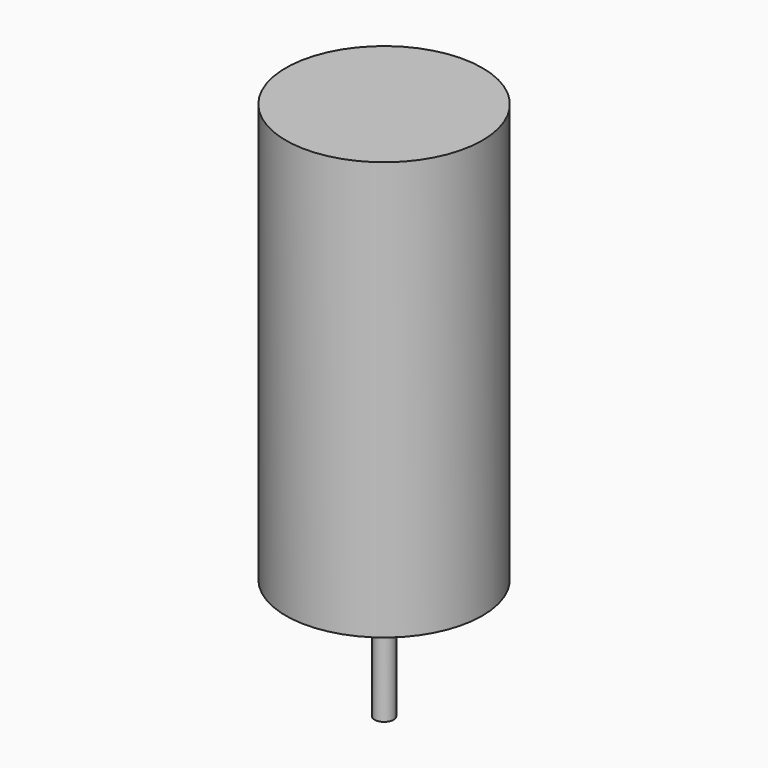
from build123d import *

# Parameters (mm, degrees)
F0_R            = 1.5
F1_DEPTH        = 19
F0_R_2          = 6
F2_DEPTH        = 3
F0_R_3          = 15.5
F3_DEPTH        = 66
F4_DEPTH        = 10
F4_COPIES_COUNT = 4


# Not quite as in the source:
# - a pattern or mirror of a feature is missing from the dataset's text; its kind, count and spacing are read off the source's solid


with BuildPart() as f1:
    # F0 (on Top) → F1 (new body)
    with BuildSketch(Plane.XY):
        Circle(F0_R)
    extrude(amount=-F1_DEPTH)

    # F0 (on Top) → F2 (join)
    with BuildSketch(Plane.XY):
        Circle(F0_R_2)
        Circle(F0_R, mode=Mode.SUBTRACT)
    extrude(amount=-F2_DEPTH)

    # F0 (on Top) → F3 (join)
    with BuildSketch(Plane.XY):
        Circle(F0_R_3)
        Circle(F0_R_2, mode=Mode.SUBTRACT)
        with Locations((7.7781745931, 7.7781745931)):
            Circle(F0_R, mode=Mode.SUBTRACT)
        Circle(F0_R_2)
        Circle(F0_R, mode=Mode.SUBTRACT)
        Circle(F0_R)
        with Locations((7.7781745931, 7.7781745931)):
            Circle(F0_R)
    extrude(amount=F3_DEPTH)

    # F0 (on Top) → F4 (cut)
    with BuildSketch(Plane.XY):
        with Locations((7.7781745931, 7.7781745931)):
            Circle(F0_R)
    f4 = extrude(amount=F4_DEPTH, mode=Mode.SUBTRACT)

    # F4_copies: F4 ×4 about axis
    f4_copies_axis = Axis((0, 0, 0), (0, 0, 1))
    for i in range(1, F4_COPIES_COUNT):
        add(f4.rotate(f4_copies_axis, i * 360 / F4_COPIES_COUNT), mode=Mode.SUBTRACT)


solid = f1.part
